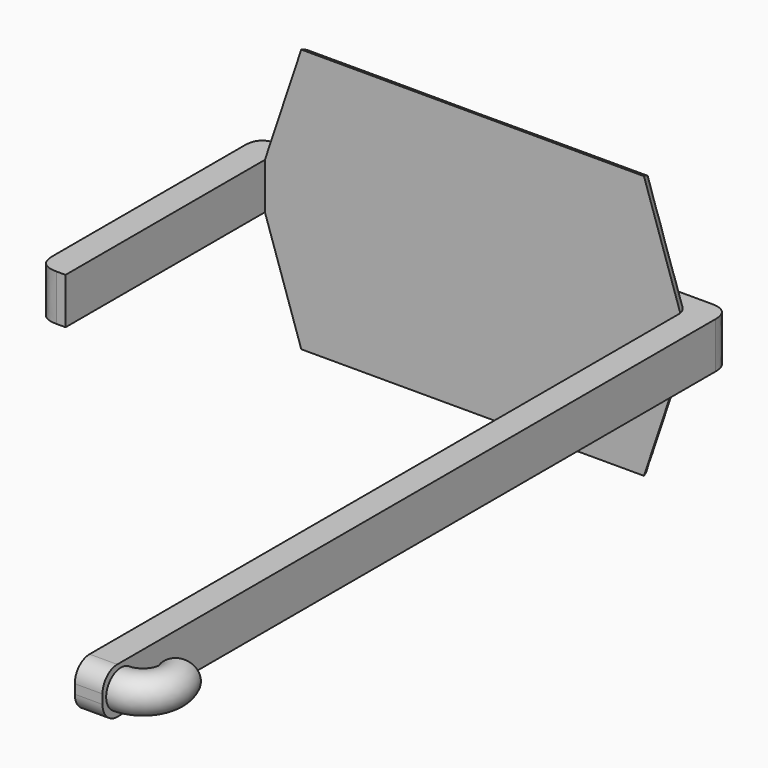
from build123d import *

# Parameters (mm, degrees)
F0_W         = 3
F0_H         = 27
F1_DEPTH     = 5
F3_DEPTH     = 1.5
F4_R         = 2
F5_ANGLE     = 116.8724050768
F6_R         = 2
F7_T1_DEPTH  = 15
F7_T3_DEPTH  = 46.8093211895
F7_T8_DEPTH  = 22.1126839652
F7_T13_DEPTH = 22.1126839652
F7_T18_DEPTH = 22.1126839652
F7_T23_DEPTH = 22.1126839652
F7_T28_DEPTH = 22.1126839652
F7_T33_DEPTH = 22.1126839652
F7_T38_DEPTH = 22.1126839652
F7_T43_DEPTH = 22.1126839652


# Not quite as in the source:
# - a fillet or chamfer that OpenCascade refuses, or shapes differently, is made with other operations: its cross-section is extruded or revolved along the edge and cut away or added


with BuildPart() as f1:
    # F0 (on Top) → F1 (new body)
    with BuildSketch(Plane.XY):
        Polygon((1.5, -42.5), (1.5, 42.5), (-1.5, 42.5), (-1.5, 39.5), (-1.5, -42.5), align=None)
        Polygon((-1.5, 39.5), (-1.5, 42.5), (-49.5, 42.5), (-49.5, 39.5), (-46.5, 39.5), align=None)
        with Locations((-48, 26)):
            Rectangle(F0_W, F0_H)
    extrude(amount=F1_DEPTH)

    # F2 (on face) → F3 (join)
    with BuildSketch(Plane.XZ.offset(-39.5)):
        Polygon((-42.563431412, 16.7904171348), (-46.5, 5), (-1.5, 5), (-5.436568588, 16.7904171348), (-24, 16.7904171348), align=None)
        Polygon((-1.5, 0), (-46.5, 0), (-42.563431412, -11.7904171348), (-24, -11.7904171348), (-5.436568588, -11.7904171348), align=None)
    extrude(amount=-F3_DEPTH)

    # F4 (on face) → F5 (revolve)
    with BuildSketch(Plane.YZ.offset(1.5)):
        with Locations((-40, 2.5)):
            Circle(F4_R)
    revolve(axis=Axis((1.5, -37, 2.371235867), (0, 0, 1)), revolution_arc=F5_ANGLE)

    # F6
    f6_edges = [f1.edges().sort_by_distance(p)[0] for p in [
        (0, -42.5, 0),
        (0, -42.5, 5),
    ]]
    fillet(f6_edges, radius=F6_R)

    # F7: fillet of radius 2 on 9 edges, made by hand

    # F7_s2 → F7_t1 (cut)
    with BuildSketch(Plane.XY.offset(-5)):
        with BuildLine():
            add(Edge.make_bspline(
                [(1.5, 40.5), (1.5, 42.5), (-0.5, 42.5)],
                knots=[0, 0, 0, 1, 1, 1], degree=2, weights=[1, 1, 1]))
            Line((-0.5, 42.5), (1.5, 42.5))
            Line((1.5, 42.5), (1.5, 40.5))
        make_face()
        with BuildLine():
            add(Edge.make_bspline(
                [(-47.5, 42.5), (-49.5, 42.5), (-49.5, 40.5)],
                knots=[0, 0, 0, 1, 1, 1], degree=2, weights=[1, 1, 1]))
            Line((-49.5, 40.5), (-49.5, 42.5))
            Line((-49.5, 42.5), (-47.5, 42.5))
        make_face()
        with BuildLine():
            add(Edge.make_bspline(
                [(-49.5, 14.5), (-49.5, 12.5), (-47.5, 12.5)],
                knots=[0, 0, 0, 1, 1, 1], degree=2, weights=[1, 1, 1]))
            Line((-47.5, 12.5), (-49.5, 12.5))
            Line((-49.5, 12.5), (-49.5, 14.5))
        make_face()
    extrude(amount=F7_T1_DEPTH, mode=Mode.SUBTRACT)

    # F7_s4 → F7_t3 (cut)
    with BuildSketch(Plane.YZ.offset(-47.4046605947)):
        with BuildLine():
            add(Edge.make_bspline(
                [(41, 14.8539254617), (41, 16.4031188001), (39.5, 16.7904171348)],
                knots=[0, 0, 0, 1, 1, 1], degree=2, weights=[1, 1, 1]))
            Line((39.5, 16.7904171348), (41, 16.7904171348))
            Line((41, 16.7904171348), (41, 14.8539254617))
        make_face()
        with BuildLine():
            add(Edge.make_bspline(
                [(41, -9.8539254617), (41, -11.4031188001), (39.5, -11.7904171348)],
                knots=[0, 0, 0, 1, 1, 1], degree=2, weights=[1, 1, 1]))
            Line((39.5, -11.7904171348), (41, -11.7904171348))
            Line((41, -11.7904171348), (41, -9.8539254617))
        make_face()
    extrude(amount=F7_T3_DEPTH, mode=Mode.SUBTRACT)


with BuildPart() as f7_tool6:
    # F7_s7 → F7_t8 (new body)
    with BuildSketch(Plane(origin=(2.3080156307, 0, 6.912737942), x_dir=(0, 1, 0), z_dir=(-0.3166932536, 0, -0.9485280086))):
        with BuildLine():
            add(Edge.make_bspline(
                [(41, -43.7535269955), (41, -45.302720334), (39.5, -45.6900186686)],
                knots=[0, 0, 0, 1, 1, 1], degree=2, weights=[1, 1, 1]))
            Line((39.5, -45.6900186686), (41, -45.6900186686))
            Line((41, -45.6900186686), (41, -43.7535269955))
        make_face()
    extrude(amount=F7_T8_DEPTH)

    split(bisect_by=Plane.XY.offset(5), keep=Keep.TOP)


with BuildPart() as f1_1:
    add(f1.part)

    # F7_t5: cut F7_tool6
    add(f7_tool6.part, mode=Mode.SUBTRACT)


with BuildPart() as f7_tool11:
    # F7_s12 → F7_t13 (new body)
    with BuildSketch(Plane(origin=(2.3080156307, 0, 6.912737942), x_dir=(0, 1, 0), z_dir=(-0.3166932536, 0, -0.9485280086))):
        with BuildLine():
            add(Edge.make_bspline(
                [(41, -43.7535269955), (41, -45.302720334), (39.5, -45.6900186686)],
                knots=[0, 0, 0, 1, 1, 1], degree=2, weights=[1, 1, 1]))
            Line((39.5, -45.6900186686), (41, -45.6900186686))
            Line((41, -45.6900186686), (41, -43.7535269955))
        make_face()
    extrude(amount=F7_T13_DEPTH)

    split(bisect_by=Plane.XY, keep=Keep.BOTTOM)


with BuildPart() as f1_2:
    add(f1_1.part)

    # F7_t10: cut F7_tool11
    add(f7_tool11.part, mode=Mode.SUBTRACT)


with BuildPart() as f7_tool16:
    # F7_s17 → F7_t18 (new body)
    with BuildSketch(Plane(origin=(-0.1192194099, 0, 0.3570740714), x_dir=(0, 1, 0), z_dir=(-0.3166932536, 0, 0.9485280086))):
        with BuildLine():
            add(Edge.make_bspline(
                [(39.5, -0.160674255), (41, 0.2266240796), (41, 1.7758174181)],
                knots=[0, 0, 0, 1, 1, 1], degree=2, weights=[1, 1, 1]))
            Line((41, 1.7758174181), (41, -0.160674255))
            Line((41, -0.160674255), (39.5, -0.160674255))
        make_face()
    extrude(amount=F7_T18_DEPTH)

    split(bisect_by=Plane.XY, keep=Keep.BOTTOM)


with BuildPart() as f1_3:
    add(f1_2.part)

    # F7_t15: cut F7_tool16
    add(f7_tool16.part, mode=Mode.SUBTRACT)


with BuildPart() as f7_tool21:
    # F7_s22 → F7_t23 (new body)
    with BuildSketch(Plane(origin=(-0.1192194099, 0, 0.3570740714), x_dir=(0, 1, 0), z_dir=(-0.3166932536, 0, 0.9485280086))):
        with BuildLine():
            add(Edge.make_bspline(
                [(39.5, -0.160674255), (41, 0.2266240796), (41, 1.7758174181)],
                knots=[0, 0, 0, 1, 1, 1], degree=2, weights=[1, 1, 1]))
            Line((41, 1.7758174181), (41, -0.160674255))
            Line((41, -0.160674255), (39.5, -0.160674255))
        make_face()
    extrude(amount=F7_T23_DEPTH)

    split(bisect_by=Plane.XY.offset(5), keep=Keep.TOP)


with BuildPart() as f1_4:
    add(f1_3.part)

    # F7_t20: cut F7_tool21
    add(f7_tool21.part, mode=Mode.SUBTRACT)


with BuildPart() as f7_tool26:
    # F7_s27 → F7_t28 (new body)
    with BuildSketch(Plane(origin=(-6.1968843057, 0, 18.5602890603), x_dir=(0, 1, 0), z_dir=(0.3166932536, 0, -0.9485280086))):
        with BuildLine():
            add(Edge.make_bspline(
                [(41, -42.1700607276), (41, -43.7192540661), (39.5, -44.1065524007)],
                knots=[0, 0, 0, 1, 1, 1], degree=2, weights=[1, 1, 1]))
            Line((39.5, -44.1065524007), (41, -44.1065524007))
            Line((41, -44.1065524007), (41, -42.1700607276))
        make_face()
    extrude(amount=F7_T28_DEPTH)

    split(bisect_by=Plane.XY.offset(5), keep=Keep.TOP)


with BuildPart() as f1_5:
    add(f1_4.part)

    # F7_t25: cut F7_tool26
    add(f7_tool26.part, mode=Mode.SUBTRACT)


with BuildPart() as f7_tool31:
    # F7_s32 → F7_t33 (new body)
    with BuildSketch(Plane(origin=(-6.1968843057, 0, 18.5602890603), x_dir=(0, 1, 0), z_dir=(0.3166932536, 0, -0.9485280086))):
        with BuildLine():
            add(Edge.make_bspline(
                [(41, -42.1700607276), (41, -43.7192540661), (39.5, -44.1065524007)],
                knots=[0, 0, 0, 1, 1, 1], degree=2, weights=[1, 1, 1]))
            Line((39.5, -44.1065524007), (41, -44.1065524007))
            Line((41, -44.1065524007), (41, -42.1700607276))
        make_face()
    extrude(amount=F7_T33_DEPTH)

    split(bisect_by=Plane.XY, keep=Keep.BOTTOM)


with BuildPart() as f1_6:
    add(f1_5.part)

    # F7_t30: cut F7_tool31
    add(f7_tool31.part, mode=Mode.SUBTRACT)


with BuildPart() as f7_tool36:
    # F7_s37 → F7_t38 (new body)
    with BuildSketch(Plane(origin=(-5.6201951346, 0, -16.8330472425), x_dir=(0, 1, 0), z_dir=(0.3166932536, 0, 0.9485280086))):
        with BuildLine():
            add(Edge.make_bspline(
                [(39.5, 1.4227920129), (41, 1.8100903475), (41, 3.359283686)],
                knots=[0, 0, 0, 1, 1, 1], degree=2, weights=[1, 1, 1]))
            Line((41, 3.359283686), (41, 1.4227920129))
            Line((41, 1.4227920129), (39.5, 1.4227920129))
        make_face()
    extrude(amount=F7_T38_DEPTH)

    split(bisect_by=Plane.XY, keep=Keep.BOTTOM)


with BuildPart() as f1_7:
    add(f1_6.part)

    # F7_t35: cut F7_tool36
    add(f7_tool36.part, mode=Mode.SUBTRACT)


with BuildPart() as f7_tool41:
    # F7_s42 → F7_t43 (new body)
    with BuildSketch(Plane(origin=(-5.6201951346, 0, -16.8330472425), x_dir=(0, 1, 0), z_dir=(0.3166932536, 0, 0.9485280086))):
        with BuildLine():
            add(Edge.make_bspline(
                [(39.5, 1.4227920129), (41, 1.8100903475), (41, 3.359283686)],
                knots=[0, 0, 0, 1, 1, 1], degree=2, weights=[1, 1, 1]))
            Line((41, 3.359283686), (41, 1.4227920129))
            Line((41, 1.4227920129), (39.5, 1.4227920129))
        make_face()
    extrude(amount=F7_T43_DEPTH)

    split(bisect_by=Plane.XY.offset(5), keep=Keep.TOP)


with BuildPart() as f1_8:
    add(f1_7.part)

    # F7_t40: cut F7_tool41
    add(f7_tool41.part, mode=Mode.SUBTRACT)


solid = f1_8.part
